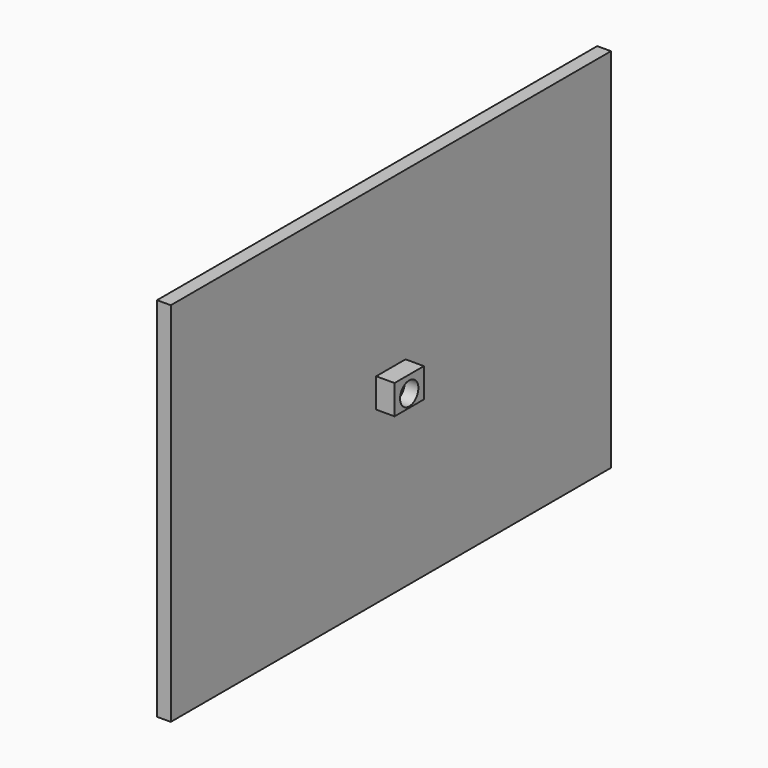
from build123d import *

# Parameters (mm, degrees)
F1_W         = 40
F1_H         = 32
F2_DEPTH     = 20
F0_W         = 600
F0_H         = 400
F3_DEPTH     = 15
F4_R         = 12.5
F5_DEPTH     = 15
F6_TEXT_SIZE = 197.7750309023
F7_DEPTH     = 5
F8_W         = 560
F8_H         = 350
F9_DEPTH     = 4


# Not quite as in the source:
# - Text() gives the source's letters only with a copy of the font that has no kerning and outlines rounded to 1/6400 em; it was checked with that copy


with BuildPart() as f2:
    # F1 (on face) → F2 (new body)
    with BuildSketch(Plane.YZ):
        with Locations((0, 2)):
            Rectangle(F1_W, F1_H)
    extrude(amount=F2_DEPTH)

    # F0 (on Right) → F3 (join)
    with BuildSketch(Plane.YZ):
        Rectangle(F0_W, F0_H)
    extrude(amount=-F3_DEPTH)

    # F4 (on face) → F5 (cut)
    with BuildSketch(Plane.YZ.offset(20)):
        Circle(F4_R)
    extrude(amount=-F5_DEPTH, mode=Mode.SUBTRACT)

    # F6 (on face) → F7 (cut)
    with BuildSketch(Plane(origin=(-15, 0, 0), x_dir=(0, -1, 0), z_dir=(-1, 0, 0))):
        with Locations((-241.1431399525, -64.7943699345)):
            Text('P.G.R', F6_TEXT_SIZE, font='Open Sans', text_align=(TextAlign.LEFT, TextAlign.BOTTOM))
    extrude(amount=-F7_DEPTH, mode=Mode.SUBTRACT)

    # F8 (on face) → F9 (cut)
    with BuildSketch(Plane(origin=(-15, 0, 0), x_dir=(0, -1, 0), z_dir=(-1, 0, 0))):
        Rectangle(F8_W, F8_H)
    extrude(amount=-F9_DEPTH, mode=Mode.SUBTRACT)


solid = f2.part
